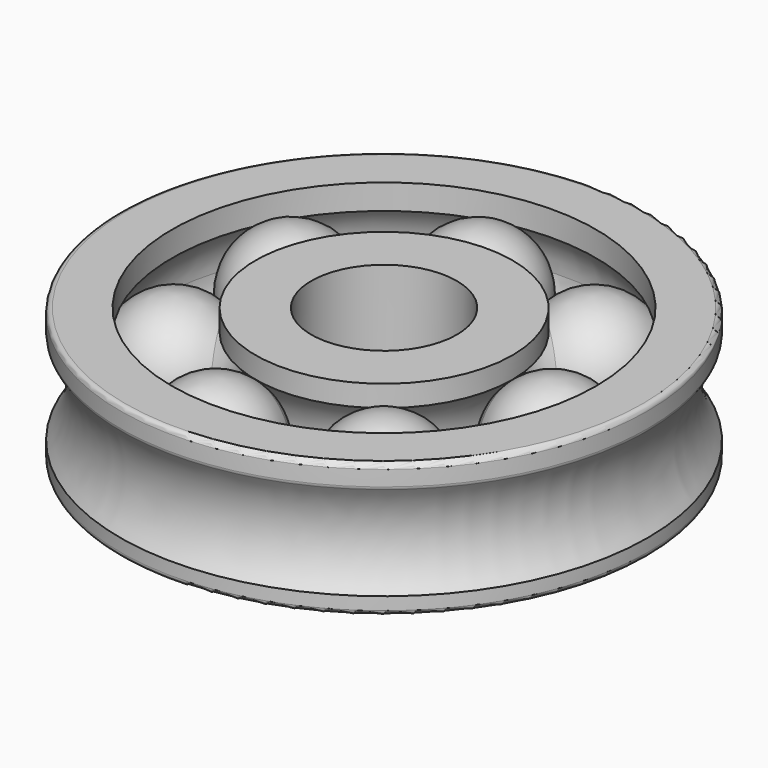
from build123d import *

# Parameters (mm, degrees)
F3_COUNT = 7
F4_R     = 1


with BuildPart() as f1:
    # F0 (on Front) → F1 (revolve)
    with BuildSketch(Plane.XZ):
        with BuildLine():
            Line((26.293175295, 13.5999182239), (14.8951485753, 13.5999182239))
            Line((14.8951485753, 13.5999182239), (14.8951485753, -12.3046878725))
            Line((14.8951485753, -12.3046878725), (26.293175295, -12.3046878725))
            Line((26.293175295, -12.3046878725), (26.293175295, -9.2098058129))
            ThreePointArc((26.293175295, -9.2098058129), (23.2323653268, -5.0497365424), (22.1484396607, 0))
            ThreePointArc((22.1484396607, 0), (23.2323653268, 5.0497365424), (26.293175295, 9.2098058129))
            Line((26.293175295, 9.2098058129), (26.293175295, 13.5999182239))
        make_face()
    revolve(axis=Axis((0, 0, 1.2304689735), (0, 0, 1)))


with BuildPart() as f1b:
    # F0 (on Front) → F1, piece 2 (revolve)
    with BuildSketch(Plane.XZ):
        with BuildLine():
            Line((43.3902144432, 13.5999182239), (43.3902144432, 8.4577669159))
            ThreePointArc((43.3902144432, 8.4577669159), (45.8849560955, 4.5517732107), (46.7578154057, 0))
            ThreePointArc((46.7578154057, 0), (45.8849560955, -4.5517732107), (43.3902144432, -8.4577669159))
            Line((43.3902144432, -8.4577669159), (43.3902144432, -13.8589646667))
            Line((43.3902144432, -13.8589646667), (54.0111064911, -13.8589646667))
            Line((54.0111064911, -13.8589646667), (54.0111064911, -10.2550508454))
            ThreePointArc((54.0111064911, -10.2550508454), (50.8185422531, -0.5688359961), (54.0111064911, 9.1173788533))
            Line((54.0111064911, 9.1173788533), (54.0111064911, 13.5999182239))
            Line((54.0111064911, 13.5999182239), (43.3902144432, 13.5999182239))
        make_face()
    revolve(axis=Axis((0, 0, 1.2304689735), (0, 0, 1)))

    # F4
    f4_edges = [f1b.edges().sort_by_distance(p)[0] for p in [
        (-54.011106, 0, 13.599918),
        (-43.390214, 0, -13.858965),
        (-54.011106, 0, -13.858965),
        (-54.011106, 0, 9.117379),
    ]]
    fillet(f4_edges, radius=F4_R)


with BuildPart() as f2:
    # F0 (on Front) → F2 (revolve)
    with BuildSketch(Plane.XZ):
        with BuildLine():
            ThreePointArc((43.3902144432, 8.4577669159), (34.9938448347, 12.2928014887), (26.293175295, 9.2098058129))
            Line((26.293175295, 9.2098058129), (26.293175295, 0))
            Line((26.293175295, 0), (43.3902144432, 0))
            Line((43.3902144432, 0), (43.3902144432, 8.4577669159))
        make_face()
        with BuildLine():
            Line((26.293175295, 0), (26.293175295, 9.2098058129))
            ThreePointArc((26.293175295, 9.2098058129), (23.2323653268, 5.0497365424), (22.1484396607, 0))
            Line((22.1484396607, 0), (26.293175295, 0))
        make_face()
        with BuildLine():
            ThreePointArc((46.7578154057, 0), (45.8849560955, 4.5517732107), (43.3902144432, 8.4577669159))
            Line((43.3902144432, 8.4577669159), (43.3902144432, 0))
            Line((43.3902144432, 0), (46.7578154057, 0))
        make_face()
    revolve(axis=Axis((34.4531275332, 0, 0), (1, 0, 0)))


with BuildPart() as f3_1:
    # F3: instance of F2
    add(f2.part.rotate(Axis((0, 0, 1.2304689735), (0, 0, 1)), 1 * 360 / F3_COUNT))


with BuildPart() as f3_2:
    # F3: instance of F2
    add(f2.part.rotate(Axis((0, 0, 1.2304689735), (0, 0, 1)), 2 * 360 / F3_COUNT))


with BuildPart() as f3_3:
    # F3: instance of F2
    add(f2.part.rotate(Axis((0, 0, 1.2304689735), (0, 0, 1)), 3 * 360 / F3_COUNT))


with BuildPart() as f3_4:
    # F3: instance of F2
    add(f2.part.rotate(Axis((0, 0, 1.2304689735), (0, 0, 1)), 4 * 360 / F3_COUNT))


with BuildPart() as f3_5:
    # F3: instance of F2
    add(f2.part.rotate(Axis((0, 0, 1.2304689735), (0, 0, 1)), 5 * 360 / F3_COUNT))


with BuildPart() as f3_6:
    # F3: instance of F2
    add(f2.part.rotate(Axis((0, 0, 1.2304689735), (0, 0, 1)), 6 * 360 / F3_COUNT))


solid = Compound([f1.part, f1b.part, f2.part, f3_1.part, f3_2.part, f3_3.part, f3_4.part, f3_5.part, f3_6.part])
